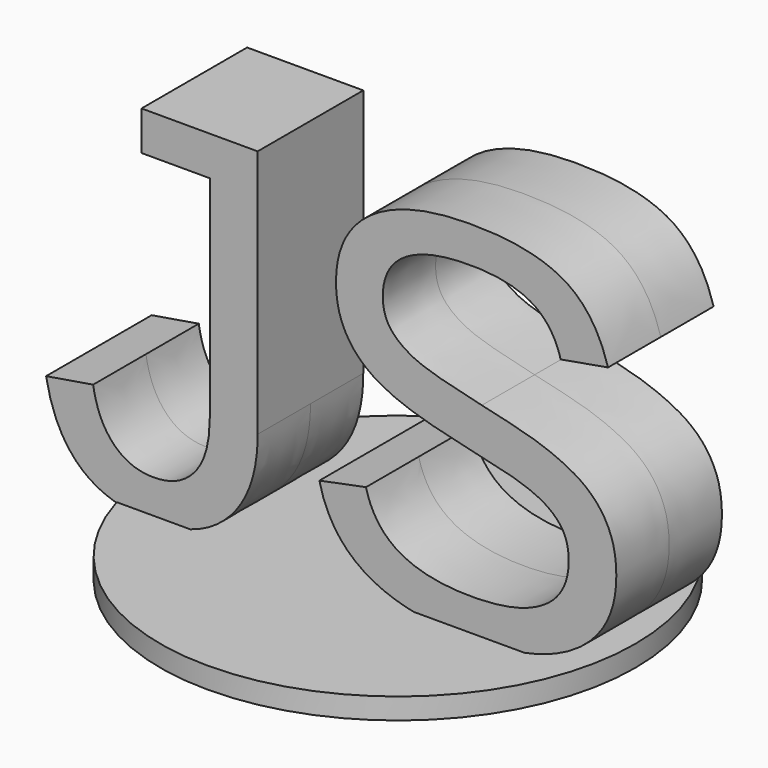
from build123d import *

# Parameters (mm, degrees)
F0_TEXT_SIZE  = 97.6952413718
F1_DEPTH      = 12.5
F4_R          = 45
F5_DEPTH      = 1
F5_DEPTH_BACK = 3


# Not quite as in the source:
# - Text() gives the source's letters only with a copy of the font that has no kerning and outlines rounded to 1/6400 em; it was checked with that copy


with BuildPart() as f1:
    # F0 (on Front) → F1 (new body, symmetric)
    with BuildSketch(Plane.XZ):
        with Locations((-58.1515659384, 0)):
            Text('JS', F0_TEXT_SIZE, font='Arimo', text_align=(TextAlign.LEFT, TextAlign.BOTTOM))
    extrude(amount=F1_DEPTH, both=True)


with BuildPart() as f5:
    # F4 (on 3pt) → F5 (new body, two sides)
    with BuildSketch(Plane.XY.offset(-0.9616875323)) as f5_sk:
        Circle(F4_R)
    extrude(amount=F5_DEPTH)
    extrude(f5_sk.sketch, amount=-F5_DEPTH_BACK)


solid = Compound([f1.part, f5.part])
